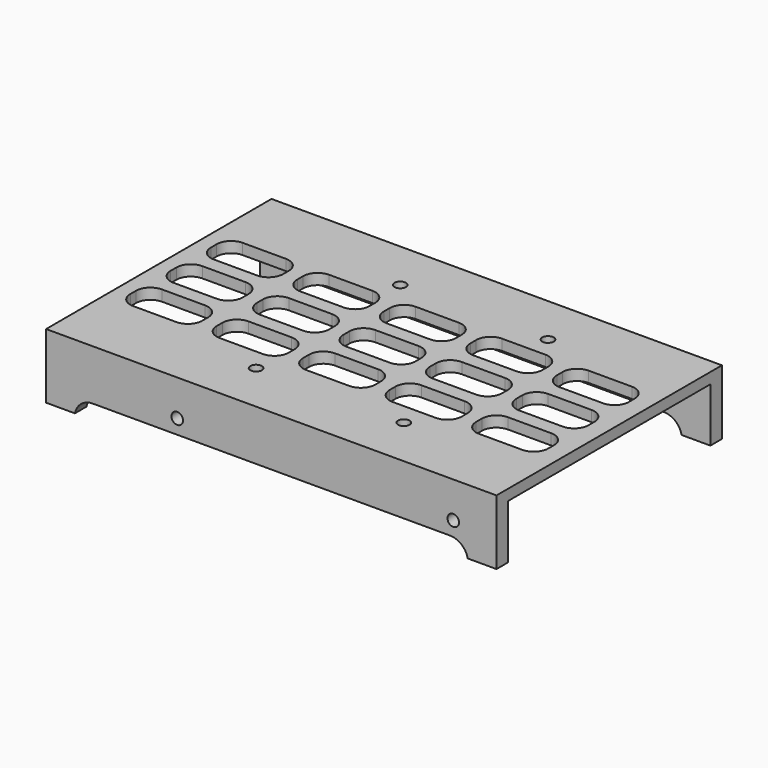
from build123d import *

# Parameters (mm, degrees)
F0_W         = 125
F0_H         = 78.2
F1_DEPTH     = 3
F2_W         = 125
F2_H         = 4
F3_DEPTH     = 15
F5_D         = 3.2
F6_W         = 109
F6_H         = 4
F7_DEPTH     = 78.201
F9_D         = 3.2
F10_T1_DEPTH = 4
F10_T3_DEPTH = 4
F12_DEPTH    = 3


# Not quite as in the source:
# - a fillet or chamfer that OpenCascade refuses, or shapes differently, is made with other operations: its cross-section is extruded or revolved along the edge and cut away or added


with BuildPart() as f1:
    # F0 (on Top) → F1 (new body)
    with BuildSketch(Plane.XY):
        with Locations((62.5, 39.1)):
            Rectangle(F0_W, F0_H)
    extrude(amount=F1_DEPTH)

    # F2 (on face) → F3 (join)
    with BuildSketch(Plane(origin=(0, 0, 0), x_dir=(1, 0, 0), z_dir=(0, 0, -1))):
        with Locations((62.5, -76.2)):
            Rectangle(F2_W, F2_H)
        with Locations((62.5, -2)):
            Rectangle(F2_W, F2_H)
    extrude(amount=F3_DEPTH)

    # F5 (through all)
    with Locations(Plane.XZ):
        with Locations((113, -7), (36.4, -7)):
            Hole(F5_D / 2)

    # F6 (on face) → F7 (cut, through all)
    with BuildSketch(Plane.XZ):
        with Locations((62.5, -13)):
            Rectangle(F6_W, F6_H)
    extrude(amount=-F7_DEPTH, mode=Mode.SUBTRACT)

    # F9 (through all)
    with Locations(Plane.XY.offset(3)):
        with Locations((47, 14.1), (88, 14.1), (88, 64.1), (47, 64.1)):
            Hole(F9_D / 2)

    # F10: fillet of radius 5 on 4 edges, made by hand

    # F10_s2 → F10_t1 (join)
    with BuildSketch(Plane.XZ.offset(-4)):
        with BuildLine():
            ThreePointArc((112.1010205144, -11), (115.2632981746, -12.1270166538), (117, -15))
            Line((117, -15), (117, -11))
            Line((117, -11), (112.1010205144, -11))
        make_face()
        with BuildLine():
            ThreePointArc((8, -15), (9.7367018254, -12.1270166538), (12.8989794856, -11))
            Line((12.8989794856, -11), (8, -11))
            Line((8, -11), (8, -15))
        make_face()
    extrude(amount=F10_T1_DEPTH)

    # F10_s4 → F10_t3 (join)
    with BuildSketch(Plane.XZ.offset(-78.2)):
        with BuildLine():
            ThreePointArc((117, -15), (115.2632981746, -12.1270166538), (112.1010205144, -11))
            Line((112.1010205144, -11), (117, -11))
            Line((117, -11), (117, -15))
        make_face()
        with BuildLine():
            ThreePointArc((12.8989794856, -11), (9.7367018254, -12.1270166538), (8, -15))
            Line((8, -15), (8, -11))
            Line((8, -11), (12.8989794856, -11))
        make_face()
    extrude(amount=F10_T3_DEPTH)

    # F11 (on face) → F12 (cut, through all)
    with BuildSketch(Plane.XY.offset(3)):
        with BuildLine():
            Line((20, 58.2), (8, 58.2))
            ThreePointArc((8, 58.2), (5.1715728753, 57.0284271247), (4, 54.2))
            Line((4, 54.2), (4, 52.2))
            ThreePointArc((4, 52.2), (5.1715728753, 49.3715728753), (8, 48.2))
            Line((8, 48.2), (20, 48.2))
            ThreePointArc((20, 48.2), (22.8284271247, 49.3715728753), (24, 52.2))
            Line((24, 52.2), (24, 54.2))
            ThreePointArc((24, 54.2), (22.8284271247, 57.0284271247), (20, 58.2))
        make_face()
        with BuildLine():
            Line((20, 44.2), (8, 44.2))
            ThreePointArc((8, 44.2), (5.1715728753, 43.0284271247), (4, 40.2))
            Line((4, 40.2), (4, 38.2))
            ThreePointArc((4, 38.2), (5.1715728753, 35.3715728753), (8, 34.2))
            Line((8, 34.2), (20, 34.2))
            ThreePointArc((20, 34.2), (22.8284271247, 35.3715728753), (24, 38.2))
            Line((24, 38.2), (24, 40.2))
            ThreePointArc((24, 40.2), (22.8284271247, 43.0284271247), (20, 44.2))
        make_face()
        with BuildLine():
            Line((20, 30.2), (8, 30.2))
            ThreePointArc((8, 30.2), (5.1715728753, 29.0284271247), (4, 26.2))
            Line((4, 26.2), (4, 24.2))
            ThreePointArc((4, 24.2), (5.1715728753, 21.3715728753), (8, 20.2))
            Line((8, 20.2), (20, 20.2))
            ThreePointArc((20, 20.2), (22.8284271247, 21.3715728753), (24, 24.2))
            Line((24, 24.2), (24, 26.2))
            ThreePointArc((24, 26.2), (22.8284271247, 29.0284271247), (20, 30.2))
        make_face()
        with BuildLine():
            Line((44, 58.2), (32, 58.2))
            ThreePointArc((32, 58.2), (29.1715728753, 57.0284271247), (28, 54.2))
            Line((28, 54.2), (28, 52.2))
            ThreePointArc((28, 52.2), (29.1715728753, 49.3715728753), (32, 48.2))
            Line((32, 48.2), (44, 48.2))
            ThreePointArc((44, 48.2), (46.8284271247, 49.3715728753), (48, 52.2))
            Line((48, 52.2), (48, 54.2))
            ThreePointArc((48, 54.2), (46.8284271247, 57.0284271247), (44, 58.2))
        make_face()
        with BuildLine():
            Line((44, 44.2), (32, 44.2))
            ThreePointArc((32, 44.2), (29.1715728753, 43.0284271247), (28, 40.2))
            Line((28, 40.2), (28, 38.2))
            ThreePointArc((28, 38.2), (29.1715728753, 35.3715728753), (32, 34.2))
            Line((32, 34.2), (44, 34.2))
            ThreePointArc((44, 34.2), (46.8284271247, 35.3715728753), (48, 38.2))
            Line((48, 38.2), (48, 40.2))
            ThreePointArc((48, 40.2), (46.8284271247, 43.0284271247), (44, 44.2))
        make_face()
        with BuildLine():
            Line((44, 30.2), (32, 30.2))
            ThreePointArc((32, 30.2), (29.1715728753, 29.0284271247), (28, 26.2))
            Line((28, 26.2), (28, 24.2))
            ThreePointArc((28, 24.2), (29.1715728753, 21.3715728753), (32, 20.2))
            Line((32, 20.2), (44, 20.2))
            ThreePointArc((44, 20.2), (46.8284271247, 21.3715728753), (48, 24.2))
            Line((48, 24.2), (48, 26.2))
            ThreePointArc((48, 26.2), (46.8284271247, 29.0284271247), (44, 30.2))
        make_face()
        with BuildLine():
            Line((68, 58.2), (56, 58.2))
            ThreePointArc((56, 58.2), (53.1715728753, 57.0284271247), (52, 54.2))
            Line((52, 54.2), (52, 52.2))
            ThreePointArc((52, 52.2), (53.1715728753, 49.3715728753), (56, 48.2))
            Line((56, 48.2), (68, 48.2))
            ThreePointArc((68, 48.2), (70.8284271247, 49.3715728753), (72, 52.2))
            Line((72, 52.2), (72, 54.2))
            ThreePointArc((72, 54.2), (70.8284271247, 57.0284271247), (68, 58.2))
        make_face()
        with BuildLine():
            Line((68, 44.2), (56, 44.2))
            ThreePointArc((56, 44.2), (53.1715728753, 43.0284271247), (52, 40.2))
            Line((52, 40.2), (52, 38.2))
            ThreePointArc((52, 38.2), (53.1715728753, 35.3715728753), (56, 34.2))
            Line((56, 34.2), (68, 34.2))
            ThreePointArc((68, 34.2), (70.8284271247, 35.3715728753), (72, 38.2))
            Line((72, 38.2), (72, 40.2))
            ThreePointArc((72, 40.2), (70.8284271247, 43.0284271247), (68, 44.2))
        make_face()
        with BuildLine():
            Line((68, 30.2), (56, 30.2))
            ThreePointArc((56, 30.2), (53.1715728753, 29.0284271247), (52, 26.2))
            Line((52, 26.2), (52, 24.2))
            ThreePointArc((52, 24.2), (53.1715728753, 21.3715728753), (56, 20.2))
            Line((56, 20.2), (68, 20.2))
            ThreePointArc((68, 20.2), (70.8284271247, 21.3715728753), (72, 24.2))
            Line((72, 24.2), (72, 26.2))
            ThreePointArc((72, 26.2), (70.8284271247, 29.0284271247), (68, 30.2))
        make_face()
        with BuildLine():
            Line((92, 58.2), (80, 58.2))
            ThreePointArc((80, 58.2), (77.1715728753, 57.0284271247), (76, 54.2))
            Line((76, 54.2), (76, 52.2))
            ThreePointArc((76, 52.2), (77.1715728753, 49.3715728753), (80, 48.2))
            Line((80, 48.2), (92, 48.2))
            ThreePointArc((92, 48.2), (94.8284271247, 49.3715728753), (96, 52.2))
            Line((96, 52.2), (96, 54.2))
            ThreePointArc((96, 54.2), (94.8284271247, 57.0284271247), (92, 58.2))
        make_face()
        with BuildLine():
            Line((92, 44.2), (80, 44.2))
            ThreePointArc((80, 44.2), (77.1715728753, 43.0284271247), (76, 40.2))
            Line((76, 40.2), (76, 38.2))
            ThreePointArc((76, 38.2), (77.1715728753, 35.3715728753), (80, 34.2))
            Line((80, 34.2), (92, 34.2))
            ThreePointArc((92, 34.2), (94.8284271247, 35.3715728753), (96, 38.2))
            Line((96, 38.2), (96, 40.2))
            ThreePointArc((96, 40.2), (94.8284271247, 43.0284271247), (92, 44.2))
        make_face()
        with BuildLine():
            Line((92, 30.2), (80, 30.2))
            ThreePointArc((80, 30.2), (77.1715728753, 29.0284271247), (76, 26.2))
            Line((76, 26.2), (76, 24.2))
            ThreePointArc((76, 24.2), (77.1715728753, 21.3715728753), (80, 20.2))
            Line((80, 20.2), (92, 20.2))
            ThreePointArc((92, 20.2), (94.8284271247, 21.3715728753), (96, 24.2))
            Line((96, 24.2), (96, 26.2))
            ThreePointArc((96, 26.2), (94.8284271247, 29.0284271247), (92, 30.2))
        make_face()
        with BuildLine():
            Line((116, 58.2), (104, 58.2))
            ThreePointArc((104, 58.2), (101.1715728753, 57.0284271247), (100, 54.2))
            Line((100, 54.2), (100, 52.2))
            ThreePointArc((100, 52.2), (101.1715728753, 49.3715728753), (104, 48.2))
            Line((104, 48.2), (116, 48.2))
            ThreePointArc((116, 48.2), (118.8284271247, 49.3715728753), (120, 52.2))
            Line((120, 52.2), (120, 54.2))
            ThreePointArc((120, 54.2), (118.8284271247, 57.0284271247), (116, 58.2))
        make_face()
        with BuildLine():
            Line((116, 44.2), (104, 44.2))
            ThreePointArc((104, 44.2), (101.1715728753, 43.0284271247), (100, 40.2))
            Line((100, 40.2), (100, 38.2))
            ThreePointArc((100, 38.2), (101.1715728753, 35.3715728753), (104, 34.2))
            Line((104, 34.2), (116, 34.2))
            ThreePointArc((116, 34.2), (118.8284271247, 35.3715728753), (120, 38.2))
            Line((120, 38.2), (120, 40.2))
            ThreePointArc((120, 40.2), (118.8284271247, 43.0284271247), (116, 44.2))
        make_face()
        with BuildLine():
            Line((116, 30.2), (104, 30.2))
            ThreePointArc((104, 30.2), (101.1715728753, 29.0284271247), (100, 26.2))
            Line((100, 26.2), (100, 24.2))
            ThreePointArc((100, 24.2), (101.1715728753, 21.3715728753), (104, 20.2))
            Line((104, 20.2), (116, 20.2))
            ThreePointArc((116, 20.2), (118.8284271247, 21.3715728753), (120, 24.2))
            Line((120, 24.2), (120, 26.2))
            ThreePointArc((120, 26.2), (118.8284271247, 29.0284271247), (116, 30.2))
        make_face()
    extrude(amount=-F12_DEPTH, mode=Mode.SUBTRACT)


solid = f1.part
